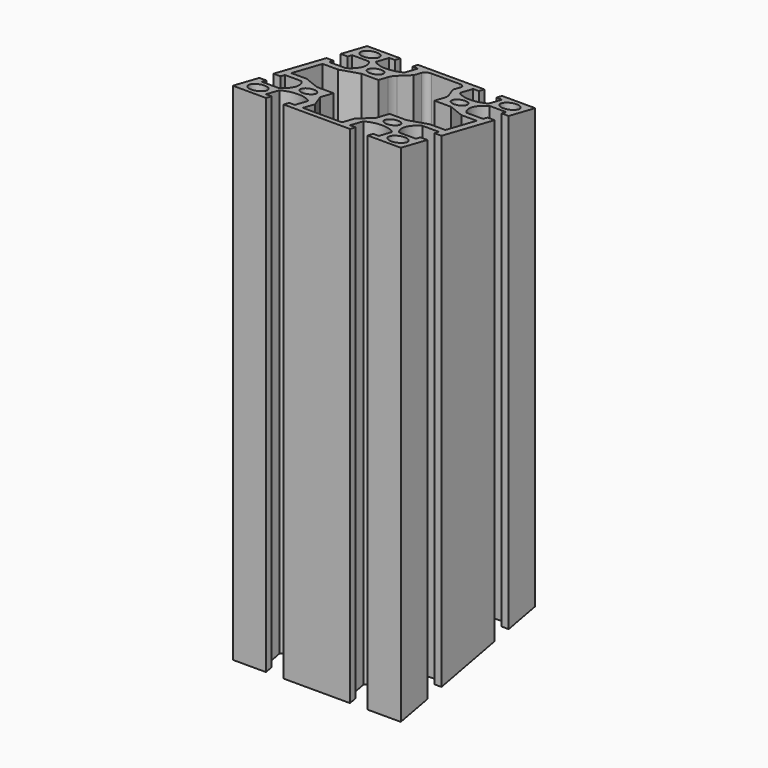
from build123d import *

# Parameters (mm, degrees)
F0_R          = 3
F0_R_2        = 2.5
F1_DEPTH      = 180.504
F2_R          = 2
F3_R          = 7
F6_DEPTH      = 30
F6_DEPTH_BACK = 30


# Not quite as in the source:
# - a feature names something its author has since deleted; it is built from what else it names


with BuildPart() as f1:
    # F0 (on Top) → F1 (new body)
    with BuildSketch(Plane.XY):
        with BuildLine():
            Line((18.15, -30), (30, -30))
            Line((30, -30), (30, -18.15))
            Line((30, -18.15), (27.5, -18.15))
            Line((27.5, -18.15), (27.5, -20.15))
            Line((27.5, -20.15), (21.5477069044, -20.15))
            ThreePointArc((21.5477069044, -20.15), (19.5, -15), (21.5477069044, -9.85))
            Line((21.5477069044, -9.85), (27.5, -9.85))
            Line((27.5, -9.85), (27.5, -11.85))
            Line((27.5, -11.85), (30, -11.85))
            Line((30, -11.85), (30, 11.85))
            Line((30, 11.85), (27.5, 11.85))
            Line((27.5, 11.85), (27.5, 9.85))
            Line((27.5, 9.85), (21.5477069044, 9.85))
            ThreePointArc((21.5477069044, 9.85), (19.5, 15), (21.5477069044, 20.15))
            Line((21.5477069044, 20.15), (27.5, 20.15))
            Line((27.5, 20.15), (27.5, 18.15))
            Line((27.5, 18.15), (30, 18.15))
            Line((30, 18.15), (30, 30))
            Line((30, 30), (18.15, 30))
            Line((18.15, 30), (18.15, 27.5))
            Line((18.15, 27.5), (20.15, 27.5))
            Line((20.15, 27.5), (20.15, 21.5477069044))
            ThreePointArc((20.15, 21.5477069044), (15, 19.5), (9.85, 21.5477069044))
            Line((9.85, 21.5477069044), (9.85, 27.5))
            Line((9.85, 27.5), (11.85, 27.5))
            Line((11.85, 27.5), (11.85, 30))
            Line((11.85, 30), (-11.85, 30))
            Line((-11.85, 30), (-11.85, 27.5))
            Line((-11.85, 27.5), (-9.85, 27.5))
            Line((-9.85, 27.5), (-9.85, 21.5477069044))
            ThreePointArc((-9.85, 21.5477069044), (-15, 19.5), (-20.15, 21.5477069044))
            Line((-20.15, 21.5477069044), (-20.15, 27.5))
            Line((-20.15, 27.5), (-18.15, 27.5))
            Line((-18.15, 27.5), (-18.15, 30))
            Line((-18.15, 30), (-30, 30))
            Line((-30, 30), (-30, 18.15))
            Line((-30, 18.15), (-27.5, 18.15))
            Line((-27.5, 18.15), (-27.5, 20.15))
            Line((-27.5, 20.15), (-21.5477069044, 20.15))
            ThreePointArc((-21.5477069044, 20.15), (-19.5, 15), (-21.5477069044, 9.85))
            Line((-21.5477069044, 9.85), (-27.5, 9.85))
            Line((-27.5, 9.85), (-27.5, 11.85))
            Line((-27.5, 11.85), (-30, 11.85))
            Line((-30, 11.85), (-30, -11.85))
            Line((-30, -11.85), (-27.5, -11.85))
            Line((-27.5, -11.85), (-27.5, -9.85))
            Line((-27.5, -9.85), (-21.5477069044, -9.85))
            ThreePointArc((-21.5477069044, -9.85), (-19.5, -15), (-21.5477069044, -20.15))
            Line((-21.5477069044, -20.15), (-27.5, -20.15))
            Line((-27.5, -20.15), (-27.5, -18.15))
            Line((-27.5, -18.15), (-30, -18.15))
            Line((-30, -18.15), (-30, -30))
            Line((-30, -30), (-18.15, -30))
            Line((-18.15, -30), (-18.15, -27.5))
            Line((-18.15, -27.5), (-20.15, -27.5))
            Line((-20.15, -27.5), (-20.15, -21.5477069044))
            ThreePointArc((-20.15, -21.5477069044), (-15, -19.5), (-9.85, -21.5477069044))
            Line((-9.85, -21.5477069044), (-9.85, -27.5))
            Line((-9.85, -27.5), (-11.85, -27.5))
            Line((-11.85, -27.5), (-11.85, -30))
            Line((-11.85, -30), (11.85, -30))
            Line((11.85, -30), (11.85, -27.5))
            Line((11.85, -27.5), (9.85, -27.5))
            Line((9.85, -27.5), (9.85, -21.5477069044))
            ThreePointArc((9.85, -21.5477069044), (15, -19.5), (20.15, -21.5477069044))
            Line((20.15, -21.5477069044), (20.15, -27.5))
            Line((20.15, -27.5), (18.15, -27.5))
            Line((18.15, -27.5), (18.15, -30))
        make_face()
        with Locations((-25, -25)):
            Circle(F0_R, mode=Mode.SUBTRACT)
        with Locations((-15, -15)):
            Circle(F0_R_2, mode=Mode.SUBTRACT)
        with Locations((25, -25)):
            Circle(F0_R, mode=Mode.SUBTRACT)
        with Locations((15, -15)):
            Circle(F0_R_2, mode=Mode.SUBTRACT)
        with Locations((-25, 25)):
            Circle(F0_R, mode=Mode.SUBTRACT)
        with Locations((-15, 15)):
            Circle(F0_R_2, mode=Mode.SUBTRACT)
        Polygon((-7, 22), (-7, 27.5), (0, 27.5), (7, 27.5), (7, 22), (10, 16), (10, 10), (16, 10), (22, 7), (27.5, 7), (27.5, 0), (27.5, -7), (22, -7), (16, -10), (10, -10), (10, -16), (7, -22), (7, -27.5), (0, -27.5), (-7, -27.5), (-7, -22), (-10, -16), (-10, -10), (-16, -10), (-22, -7), (-27.5, -7), (-27.5, 0), (-27.5, 7), (-22, 7), (-16, 10), (-10, 10), (-10, 16), align=None, mode=Mode.SUBTRACT)
        with Locations((15, 15)):
            Circle(F0_R_2, mode=Mode.SUBTRACT)
        with Locations((25, 25)):
            Circle(F0_R, mode=Mode.SUBTRACT)
    extrude(amount=F1_DEPTH)

    # F2
    f2_edges = [f1.edges().sort_by_distance(p)[0] for p in [
        (-7, 27.5, 90.252),
        (7, 27.5, 90.252),
    ]]
    fillet(f2_edges, radius=F2_R)

    # F3
    f3_edges = [f1.edges().sort_by_distance(p)[0] for p in [
        (-10, 16, 90.252),
        (10, 16, 90.252),
    ]]
    fillet(f3_edges, radius=F3_R)

    # F5 (on Right) → F6 (cut, two sides)
    with BuildSketch(Plane.YZ) as f6_sk:
        Polygon((166.5976946582, -66.7170951811), (146.3493769552, 35.0780720561), (-30, 0), (-9.751682297, -101.7951672372), align=None)
        Polygon((135.5963626007, 147.5648354856), (151.7094622056, 228.5708574701), (-13.8869003951, 261.5100219845), (-30, 180.504), align=None)
    extrude(amount=F6_DEPTH, mode=Mode.SUBTRACT)
    extrude(f6_sk.sketch, amount=-F6_DEPTH_BACK, mode=Mode.SUBTRACT)


solid = f1.part
